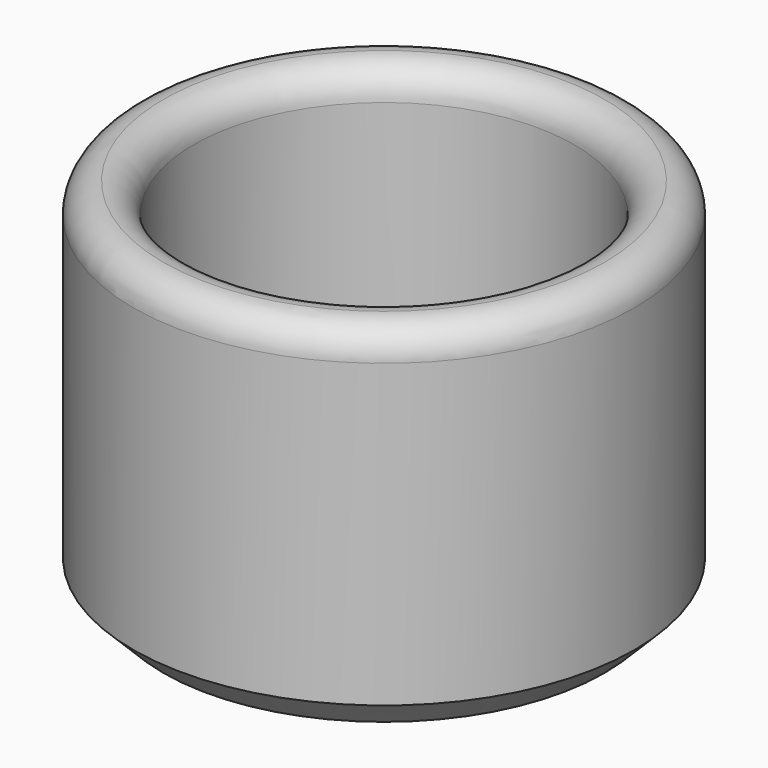
from build123d import *

# Parameters (mm, degrees)
F0_R     = 16.65
F0_R_2   = 12.65
F1_DEPTH = 20
F2_DEPTH = 4
F3_SIZE  = 2
F4_R     = 1.99999


# Not quite as in the source:
# - a fillet or chamfer is up to 0.001 mm smaller than in the source, because OpenCascade refuses the exact size


with BuildPart() as f1:
    # F0 (on Top) → F1 (new body)
    with BuildSketch(Plane.XY):
        Circle(F0_R)
        Circle(F0_R_2, mode=Mode.SUBTRACT)
    extrude(amount=F1_DEPTH)

    # F0 (on Top) → F2 (join)
    with BuildSketch(Plane.XY):
        Circle(F0_R)
        Circle(F0_R_2, mode=Mode.SUBTRACT)
        Circle(F0_R_2)
    extrude(amount=-F2_DEPTH)

    # F3
    f3_edges = [f1.edges().sort_by_distance(p)[0] for p in [
        (-16.65, 0, -4),
    ]]
    chamfer(f3_edges, length=F3_SIZE)

    # F4 (radius 2 in the source; OpenCascade refuses exactly that, so slightly less here)
    f4_edges = [f1.edges().sort_by_distance(p)[0] for p in [
        (-12.65, 0, 20),
        (-16.65, 0, 20),
    ]]
    fillet(f4_edges, radius=F4_R)


solid = f1.part
